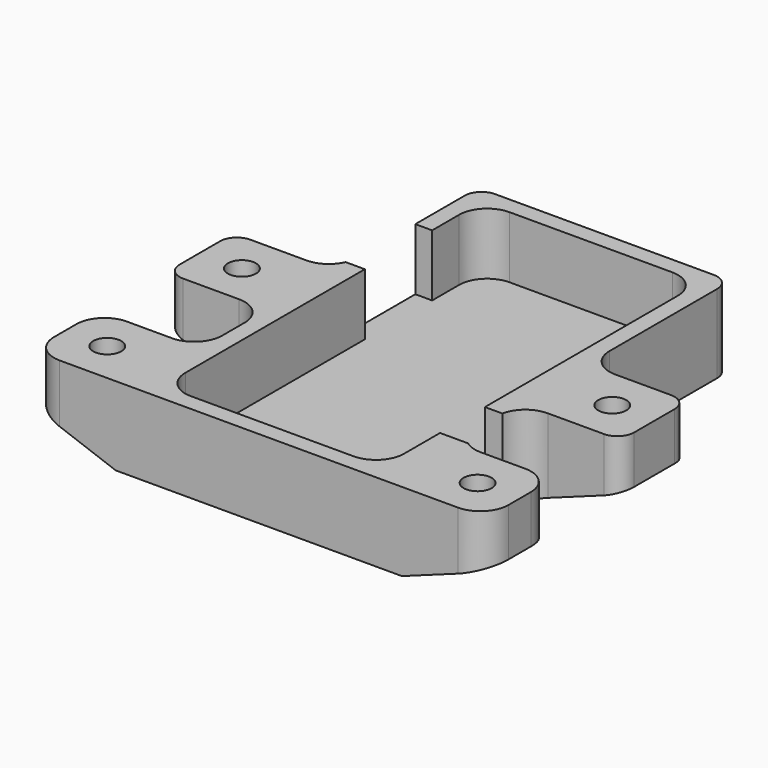
from build123d import *

# Parameters (mm, degrees)
F0_W      = 45
F0_H      = 77
F1_DEPTH  = 3
F4_DEPTH  = 11
F5_W      = 18
F5_H      = 15
F5_R      = 2.5
F6_DEPTH  = 14
F7_R      = 3
F8_R      = 5
F9_R      = 5
F11_DEPTH = 77.001


# Not quite as in the source:
# - a feature names something its author has since deleted; it is built from what else it names


with BuildPart() as f1:
    # F0 (on Top) → F1 (new body)
    with BuildSketch(Plane.XY):
        Rectangle(F0_W, F0_H)
    extrude(amount=F1_DEPTH)

    # F3 (on face) → F4 (join)
    with BuildSketch(Plane.XY.offset(3)):
        Polygon((19.5, -12.5), (22.5, -12.5), (22.5, 38.5), (-22.5, 38.5), (-22.5, 24.5), (-19.5, 24.5), (-19.5, 35.5), (19.5, 35.5), align=None)
        Polygon((22.5, -38.5), (22.5, -22.5), (19.5, -22.5), (19.5, -22.7520468089), (19.5, -35.5), (-19.5, -35.5), (-19.5, 9.5), (-22.5, 9.5), (-22.5, -38.5), align=None)
    extrude(amount=F4_DEPTH)

    # F5 (on Top) → F6 (join, through all)
    with BuildSketch(Plane.XY):
        with Locations((31.5, -1)):
            Rectangle(F5_W, F5_H)
        with Locations((33, -1)):
            Circle(F5_R, mode=Mode.SUBTRACT)
        with Locations((-31.5, -31)):
            Rectangle(F5_W, F5_H)
        with Locations((-33, -31)):
            Circle(F5_R, mode=Mode.SUBTRACT)
        with Locations((-31.5, -1)):
            Rectangle(F5_W, F5_H)
        with Locations((-33, -1)):
            Circle(F5_R, mode=Mode.SUBTRACT)
        with Locations((31.5, -31)):
            Rectangle(F5_W, F5_H)
        with Locations((33, -31)):
            Circle(F5_R, mode=Mode.SUBTRACT)
    extrude(amount=F6_DEPTH)

    # F7
    f7_edges = [f1.edges().sort_by_distance(p)[0] for p in [
        (-22.5, 38.5, 7),
        (22.5, 38.5, 7),
        (40.5, 6.5, 7),
        (40.5, -8.5, 7),
        (-40.5, 6.5, 7),
        (-40.5, -8.5, 7),
    ]]
    fillet(f7_edges, radius=F7_R)

    # F8
    f8_edges = [f1.edges().sort_by_distance(p)[0] for p in [
        (19.5, -35.5, 8.5),
        (-19.5, -35.5, 8.5),
        (19.5, 35.5, 8.5),
        (-19.5, 35.5, 8.5),
        (22.5, 6.5, 7),
        (22.5, -8.5, 7),
        (-22.5, -8.5, 7),
        (-22.5, 6.5, 7),
    ]]
    fillet(f8_edges, radius=F8_R)

    # F9
    f9_edges = [f1.edges().sort_by_distance(p)[0] for p in [
        (-40.5, -23.5, 7),
        (-22.5, -23.5, 7),
        (-40.5, -38.5, 7),
        (40.5, -38.5, 7),
        (40.5, -23.5, 7),
        (22.5, -23.5, 7),
    ]]
    fillet(f9_edges, radius=F9_R)

    # F10 (on face) → F11 (cut, through all)
    with BuildSketch(Plane.XZ.offset(38.5)):
        Polygon((-35.5, 0), (-25.5, 0), (-35.5, 3.6397023427), align=None)
        Polygon((-35.5, 0), (-35.5, 3.6397023427), (-49.4253699631, 8.7081225104), (-49.4253699631, 0), align=None)
        Polygon((35.5, 3.6397023427), (25.5, 0), (35.5, 0), align=None)
        Polygon((46.6463356366, 7.6966367355), (35.5, 3.6397023427), (35.5, 0), (46.6463356366, 0), align=None)
    extrude(amount=-F11_DEPTH, mode=Mode.SUBTRACT)


solid = f1.part
